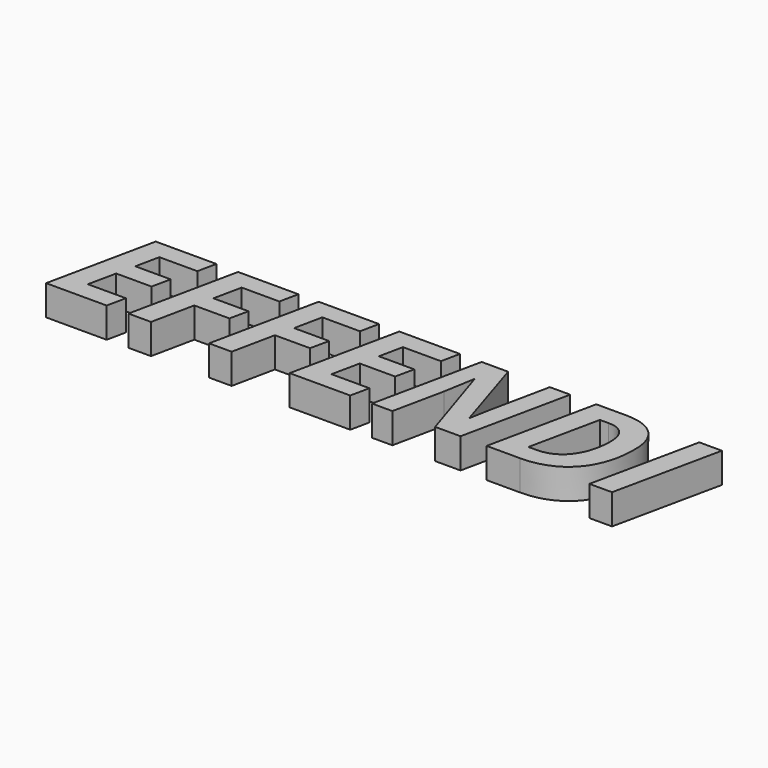
from build123d import *

# Parameters (mm, degrees)
F0_TEXT_SIZE = 25.1938747392
F1_DEPTH     = 5


# Not quite as in the source:
# - Text() gives the source's letters only with a copy of the font that has no kerning and outlines rounded to 1/6400 em; it was checked with that copy


with BuildPart() as f1:
    # F0 (on Top) → F1 (new body)
    with BuildSketch(Plane.XY):
        with Locations((-42.4062313687, -8.4275084938)):
            Text('EFFENDI', F0_TEXT_SIZE, font='Open Sans', font_style=FontStyle.BOLDITALIC, text_align=(TextAlign.LEFT, TextAlign.BOTTOM))
    extrude(amount=F1_DEPTH)


solid = f1.part
